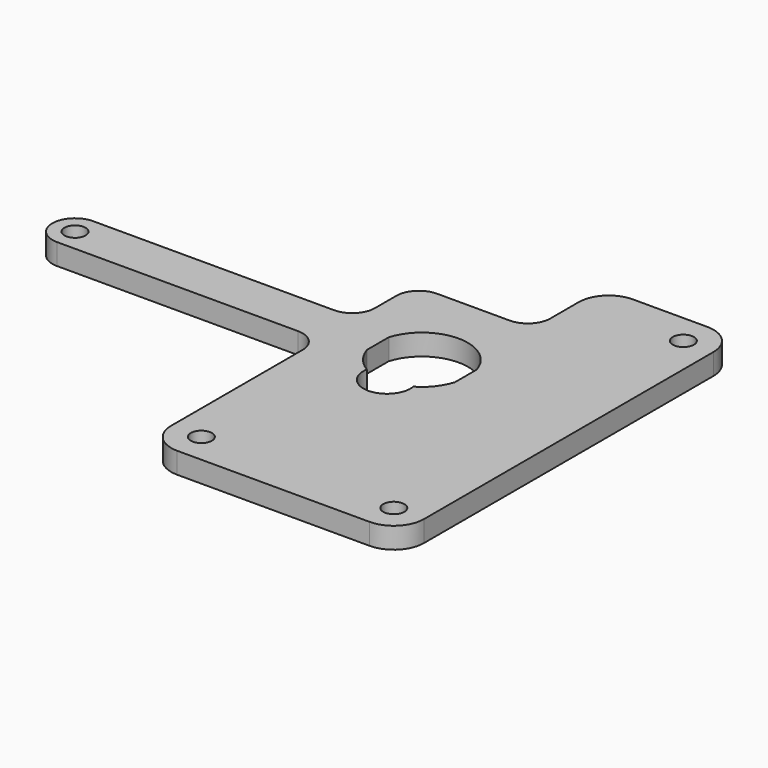
from build123d import *

# Parameters (mm, degrees)
F0_W     = 11.65
F0_H     = 23.75
F1_DEPTH = 20.4
F3_DEPTH = 6
F5_START = -0.8
F4_W     = 11.65
F4_H     = 4.2
F5_DEPTH = 2
F6_R     = 0.5
F7_R     = 1
F8_R     = 1.4
F9_DEPTH = 2.8
F10_R    = 4


# Not quite as in the source:
# - a feature names something its author has since deleted; it is built from what else it names


with BuildPart() as f1:
    # F0 (on Top) → F1 (new body)
    with BuildSketch(Plane.XY):
        Rectangle(F0_W, F0_H)
    extrude(amount=F1_DEPTH)

    # F2 (on face) → F3 (join)
    with BuildSketch(Plane.XY.offset(20.4)):
        with BuildLine():
            Line((5.825, 3.9640955299), (5.825, 7.5859044701))
            ThreePointArc((5.825, 7.5859044701), (0, 11.875), (-5.825, 7.5859044701))
            Line((-5.825, 7.5859044701), (-5.825, 3.9640955299))
            ThreePointArc((-5.825, 3.9640955299), (-4.7781429098, 1.9829886164), (-3.0865775367, 0.5135326087))
            ThreePointArc((-3.0865775367, 0.5135326087), (0, -3.1), (3.0865775367, 0.5135326087))
            ThreePointArc((3.0865775367, 0.5135326087), (4.7781429098, 1.9829886164), (5.825, 3.9640955299))
        make_face()
    extrude(amount=F3_DEPTH)

    # F4 (on face) → F5 (join)
    with BuildSketch(Plane.XY.offset(20.4).offset(F5_START)):
        with Locations((0, -13.975)):
            Rectangle(F4_W, F4_H)
        with Locations((0, 13.975)):
            Rectangle(F4_W, F4_H)
    extrude(amount=-F5_DEPTH)

    # F6
    f6_edges = [f1.edges().sort_by_distance(p)[0] for p in [
        (5.825, 11.875, 8.8),
        (5.825, -11.875, 8.8),
        (-5.825, -11.875, 8.8),
        (-5.825, 11.875, 8.8),
    ]]
    fillet(f6_edges, radius=F6_R)

    # F7
    f7_edges = [f1.edges().sort_by_distance(p)[0] for p in [
        (-5.825, 16.075, 18.6),
        (5.825, 16.075, 18.6),
        (5.825, -16.075, 18.6),
        (-5.825, -16.075, 18.6),
    ]]
    fillet(f7_edges, radius=F7_R)


with BuildPart() as f9:
    # F8 (on face) → F9 (new body)
    with BuildSketch(Plane.XY.offset(26.4)):
        with BuildLine():
            Line((22.5, -26), (22.5, 30))
            Line((22.5, 30), (4.6129450202, 30))
            Line((4.6129450202, 30), (4.6129450202, 21.3236394078))
            ThreePointArc((4.6129450202, 21.3236394078), (3.7342653638, 19.2023190642), (1.6129450202, 18.3236394078))
            Line((1.6129450202, 18.3236394078), (-8.0251465812, 18.3236394078))
            ThreePointArc((-8.0251465812, 18.3236394078), (-10.1464669248, 17.4449597513), (-11.0251465812, 15.3236394078))
            Line((-11.0251465812, 15.3236394078), (-11.0251465812, 11.775))
            ThreePointArc((-11.0251465812, 11.775), (-11.9038262377, 9.6536796564), (-14.0251465812, 8.775))
            Line((-14.0251465812, 8.775), (-46, 8.775))
            ThreePointArc((-46, 8.775), (-49, 5.775), (-46, 2.775))
            Line((-46, 2.775), (-14.0251465812, 2.775))
            ThreePointArc((-14.0251465812, 2.775), (-11.9038262377, 1.8963203436), (-11.0251465812, -0.225))
            Line((-11.0251465812, -0.225), (-11.0251465812, -15.0673655123))
            Line((-11.0251465812, -15.0673655123), (-11.0251465812, -26))
            Line((-11.0251465812, -26), (22.5, -26))
        make_face()
        with Locations((-7.0251465812, -22)):
            Circle(F8_R, mode=Mode.SUBTRACT)
        with Locations((18.5, -22)):
            Circle(F8_R, mode=Mode.SUBTRACT)
        with Locations((-46, 5.775)):
            Circle(F8_R, mode=Mode.SUBTRACT)
        with BuildLine():
            ThreePointArc((5.825, 3.9640955299), (4.7781429098, 1.9829886164), (3.0865775367, 0.5135326087))
            ThreePointArc((3.0865775367, 0.5135326087), (0, -3.1290056936), (-3.0865775367, 0.5135326087))
            ThreePointArc((-3.0865775367, 0.5135326087), (-4.7781429098, 1.9829886164), (-5.825, 3.9640955299))
            Line((-5.825, 3.9640955299), (-5.825, 7.5859044701))
            ThreePointArc((-5.825, 7.5859044701), (0, 11.875), (5.825, 7.5859044701))
            Line((5.825, 7.5859044701), (5.825, 3.9640955299))
        make_face(mode=Mode.SUBTRACT)
        with Locations((18.5, 26)):
            Circle(F8_R, mode=Mode.SUBTRACT)
    extrude(amount=-F9_DEPTH)

    # F10
    f10_edges = [f9.edges().sort_by_distance(p)[0] for p in [
        (22.5, 30, 25),
        (-11.025147, -26, 25),
        (22.5, -26, 25),
        (4.612945, 30, 25),
    ]]
    fillet(f10_edges, radius=F10_R)


with BuildPart() as f11_1:
    # F11: copy of F9
    add(f9.part)


solid = f9.part
